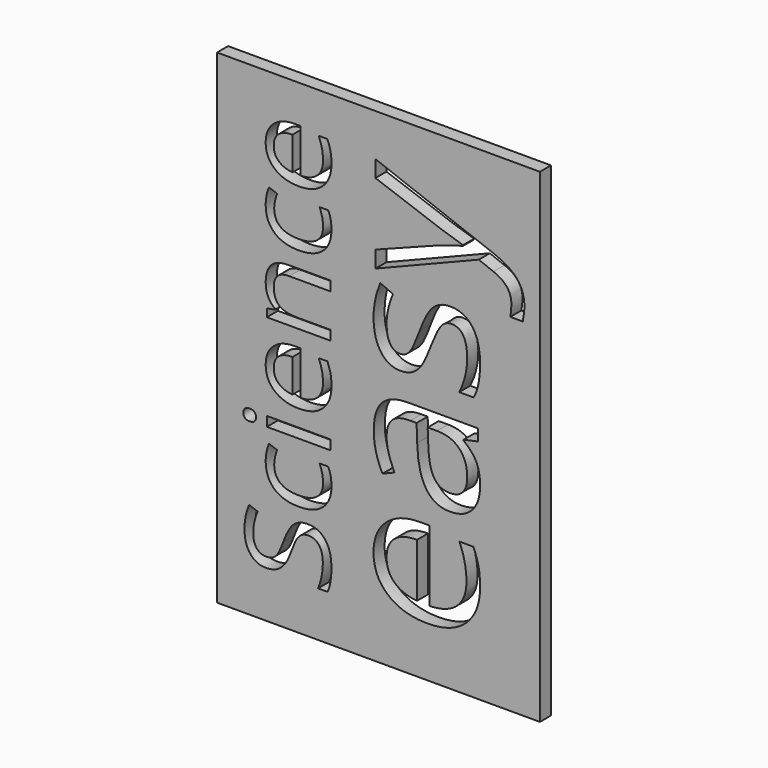
from build123d import *

# Parameters (mm, degrees)
F0_W           = 70
F0_H           = 105
F1_DEPTH       = 3
F2_TEXT_SIZE   = 25.6959314775
F2_TEXT_SIZE_2 = 41.6275204163
F3_DEPTH       = 25.4


# Not quite as in the source:
# - Text() gives the source's letters only with a copy of the font that has no kerning and outlines rounded to 1/6400 em; it was checked with that copy


with BuildPart() as f1:
    # F0 (on Front) → F1 (new body)
    with BuildSketch(Plane.XZ):
        with Locations((35, 52.5)):
            Rectangle(F0_W, F0_H)
    extrude(amount=F1_DEPTH)

    # F2 (on face) → F3 (cut)
    with BuildSketch(Plane.XZ.offset(3)):
        with Locations(Location((24.5551364625, 8.5234189758), (0, 0, 90))):
            Text('Science', F2_TEXT_SIZE, font='Open Sans', text_align=(TextAlign.LEFT, TextAlign.BOTTOM))
        with Locations(Location((56.6197829174, 8.5234189758), (0, 0, 90))):
            Text('easy', F2_TEXT_SIZE_2, font='Open Sans', text_align=(TextAlign.LEFT, TextAlign.BOTTOM))
    extrude(amount=-F3_DEPTH, mode=Mode.SUBTRACT)


solid = f1.part
